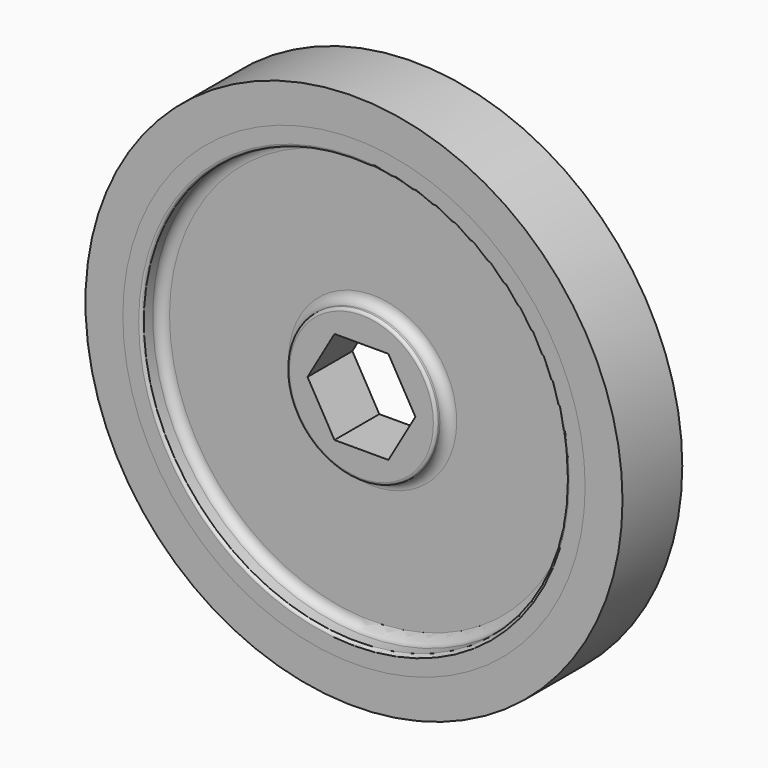
from build123d import *

# Parameters (mm, degrees)
F0_W     = 18.7325
F0_H     = 1.905
F0_W_2   = 2.54
F0_H_2   = 2.54
F3_DEPTH = 8.891
F8_R     = 1.27
F9_R     = 0.381
F10_R    = 0.381
F11_R    = 0.381


# Not quite as in the source:
# - a variable given as a bare number and used for a length is read in inches; the dataset says mm whatever the document's units were


with BuildPart() as f1:
    # F0 (on Top) → F1 (revolve)
    with BuildSketch(Plane.XY):
        Polygon((0, 3.81), (0, 0), (10.16, 0), (10.16, 1.905), (10.16, 3.81), align=None)
        with Locations((19.52625, 0.9525)):
            Rectangle(F0_W, F0_H)
        Polygon((10.16, 0), (0, 0), (0, -3.81), (10.16, -3.81), (10.16, -1.905), align=None)
        with Locations((19.52625, -0.9525)):
            Rectangle(F0_W, F0_H)
        with Locations((32.7025, -1.27)):
            Rectangle(F0_W_2, F0_H_2)
        with Locations((32.7025, 1.27)):
            Rectangle(F0_W_2, F0_H_2)
        Polygon((28.8925, 1.905), (28.8925, 0), (31.4325, 0), (31.4325, 2.54), (31.4325, 5.08), (28.8925, 5.08), align=None)
        Polygon((31.4325, 0), (28.8925, 0), (28.8925, -1.905), (28.8925, -5.08), (31.4325, -5.08), (31.4325, -2.54), align=None)
    revolve(axis=Axis((0, 1.905, 0), (0, 1, 0)))

    # F2 (on face) → F3 (cut, through all)
    with BuildSketch(Plane.XZ.offset(3.81)):
        Polygon((3.6661742094, 6.35), (-3.6661742094, 6.35), (-7.3323484187, 0), (-3.6661742094, -6.35), (3.6661742094, -6.35), (7.3323484187, 0), align=None)
    extrude(amount=-F3_DEPTH, mode=Mode.SUBTRACT)

    # F8
    f8_edges = [f1.edges().sort_by_distance(p)[0] for p in [
        (-28.8925, -1.905, 0),
        (-10.16, -1.905, 0),
        (-28.8925, 1.905, 0),
        (-10.16, 1.905, 0),
    ]]
    fillet(f8_edges, radius=F8_R)

    # F9
    f9_edges = [f1.edges().sort_by_distance(p)[0] for p in [
        (-28.8925, -5.08, 0),
        (-10.16, -3.81, 0),
    ]]
    fillet(f9_edges, radius=F9_R)

    # F10
    f10_edges = [f1.edges().sort_by_distance(p)[0] for p in [
        (-31.4325, -2.54, 0),
        (-33.9725, -2.54, 0),
        (-31.4325, 2.54, 0),
        (-33.9725, 2.54, 0),
    ]]
    fillet(f10_edges, radius=F10_R)


with BuildPart() as f5:
    # F4 (on Top) → F5 (revolve)
    with BuildSketch(Plane.XY):
        Polygon((31.4325, 5.08), (31.4325, 2.54), (33.9725, 2.54), (33.9725, 0), (33.9725, -2.54), (31.4325, -2.54), (31.4325, -5.08), (36.5125, -5.08), (36.5125, 5.08), align=None)
    revolve(axis=Axis((0, 1.905, 0), (0, 1, 0)))

    # F11
    f11_edges = [f5.edges().sort_by_distance(p)[0] for p in [
        (-33.9725, 2.54, 0),
        (-31.4325, 2.54, 0),
        (-31.4325, -2.54, 0),
        (-33.9725, -2.54, 0),
    ]]
    fillet(f11_edges, radius=F11_R)


solid = Compound([f1.part, f5.part])
